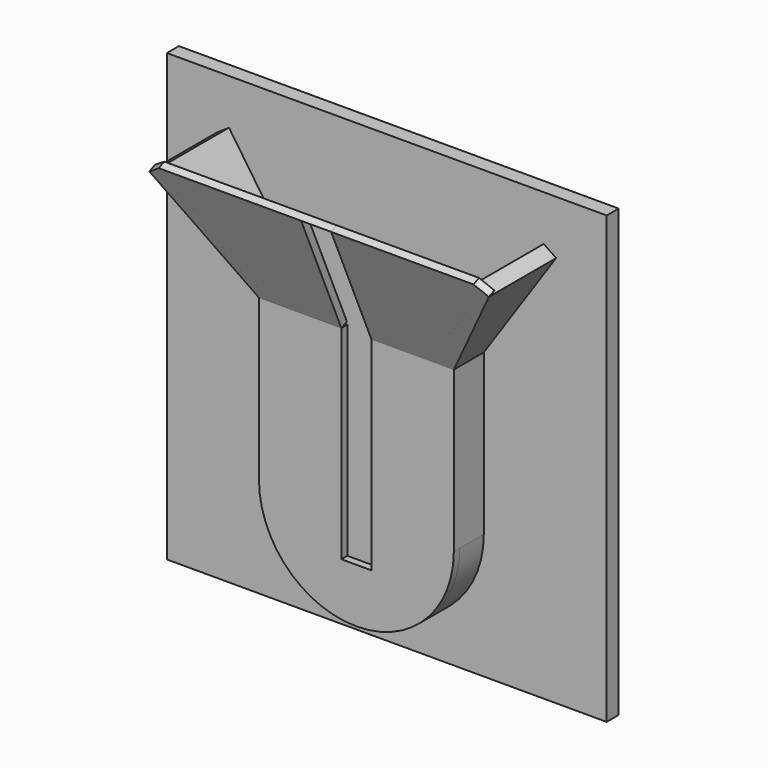
from build123d import *

# Parameters (mm, degrees)
F1_DEPTH     = 50.8
F2_W         = 745.3036904335
F2_H         = 755.5955052376
F3_DEPTH     = 25.4
F5_DEPTH     = 12.7
F7_DEPTH     = 101.6
F8_T4_DEPTH  = 1078.7585913979
F9_DEPTH     = 101.6
F10_T4_DEPTH = 1078.7585913979
F12_DEPTH    = 12.7


# Not quite as in the source:
# - a fillet or chamfer that OpenCascade refuses, or shapes differently, is made with other operations: its cross-section is extruded or revolved along the edge and cut away or added


with BuildPart() as f1:
    # F0 (on Front) → F1 (new body)
    with BuildSketch(Plane.XZ):
        with BuildLine():
            Line((-89.9567651826, 106.8080672332), (-216.9567651826, 293.8318768854))
            Line((-216.9567651826, 293.8318768854), (-237.969898878, 279.5627419326))
            Line((-237.969898878, 279.5627419326), (-216.9567651826, 248.6182040079))
            Line((-216.9567651826, 248.6182040079), (-115.3567651826, 98.9991562862))
            Line((-115.3567651826, 98.9991562862), (-115.3567651826, -172.5919327668))
            ThreePointArc((-115.3567651826, -172.5919327668), (-67.0000946798, -289.3352624173), (49.7432350342, -337.6919327668))
            ThreePointArc((49.7432350342, -337.6919327668), (166.486564468, -289.335262264), (214.8432348174, -172.5919327668))
            Line((214.8432348174, -172.5919327668), (214.8432348174, 98.9991562862))
            Line((214.8432348174, 98.9991562862), (316.4432348174, 248.6182040079))
            Line((316.4432348174, 248.6182040079), (337.4563685128, 279.5627419326))
            Line((337.4563685128, 279.5627419326), (316.4432348174, 293.8318768854))
            Line((316.4432348174, 293.8318768854), (189.4432348174, 106.8080672332))
            Line((189.4432348174, 106.8080672332), (189.4432348174, -172.5919327668))
            ThreePointArc((189.4432348174, -172.5919327668), (49.7432348174, -312.2919327668), (-89.9567651826, -172.5919327668))
            Line((-89.9567651826, -172.5919327668), (-89.9567651826, 106.8080672332))
        make_face()
    extrude(amount=F1_DEPTH)

    # F2 (on face) → F3 (join)
    with BuildSketch(Plane(origin=(0, 0, 0), x_dir=(-1, 0, 0), z_dir=(0, 1, 0))):
        with Locations((-50.4573881626, -6.8071186543)):
            Rectangle(F2_W, F2_H)
        with BuildLine():
            Line((89.9567651826, 106.8080672332), (216.9567651826, 293.8318768854))
            Line((216.9567651826, 293.8318768854), (237.969898878, 279.5627419326))
            Line((237.969898878, 279.5627419326), (115.3567651826, 98.9991562862))
            Line((115.3567651826, 98.9991562862), (115.3567651826, -172.5919327668))
            ThreePointArc((115.3567651826, -172.5919327668), (-49.7432348174, -337.6919327668), (-214.8432348174, -172.5919327668))
            Line((-214.8432348174, -172.5919327668), (-214.8432348174, 98.9991562862))
            Line((-214.8432348174, 98.9991562862), (-337.4563685128, 279.5627419326))
            Line((-337.4563685128, 279.5627419326), (-316.4432348174, 293.8318768854))
            Line((-316.4432348174, 293.8318768854), (-189.4432348174, 106.8080672332))
            Line((-189.4432348174, 106.8080672332), (-189.4432348174, -172.5919327668))
            ThreePointArc((-189.4432348174, -172.5919327668), (-49.7432348174, -312.2919327668), (89.9567651826, -172.5919327668))
            Line((89.9567651826, -172.5919327668), (89.9567651826, 106.8080672332))
        make_face(mode=Mode.SUBTRACT)
        with BuildLine():
            Line((237.969898878, 279.5627419326), (216.9567651826, 293.8318768854))
            Line((216.9567651826, 293.8318768854), (89.9567651826, 106.8080672332))
            Line((89.9567651826, 106.8080672332), (89.9567651826, -172.5919327668))
            ThreePointArc((89.9567651826, -172.5919327668), (-49.7432348174, -312.2919327668), (-189.4432348174, -172.5919327668))
            Line((-189.4432348174, -172.5919327668), (-189.4432348174, 106.8080672332))
            Line((-189.4432348174, 106.8080672332), (-316.4432348174, 293.8318768854))
            Line((-316.4432348174, 293.8318768854), (-337.4563685128, 279.5627419326))
            Line((-337.4563685128, 279.5627419326), (-214.8432348174, 98.9991562862))
            Line((-214.8432348174, 98.9991562862), (-214.8432348174, -172.5919327668))
            ThreePointArc((-214.8432348174, -172.5919327668), (-49.7432348174, -337.6919327668), (115.3567651826, -172.5919327668))
            Line((115.3567651826, -172.5919327668), (115.3567651826, 98.9991562862))
            Line((115.3567651826, 98.9991562862), (237.969898878, 279.5627419326))
        make_face()
    extrude(amount=F3_DEPTH)

    # F4 (on face) → F5 (join)
    with BuildSketch(Plane.XZ.offset(50.8)):
        with BuildLine():
            Line((24.3432348174, 98.9991562862), (-89.9567651826, 98.9991562862))
            Line((-89.9567651826, 98.9991562862), (-89.9567651826, -172.5919327668))
            ThreePointArc((-89.9567651826, -172.5919327668), (49.7432348174, -312.2919327668), (189.4432348174, -172.5919327668))
            Line((189.4432348174, -172.5919327668), (189.4432348174, 98.9991562862))
            Line((189.4432348174, 98.9991562862), (75.1432348174, 98.9991562862))
            Line((75.1432348174, 98.9991562862), (75.1432348174, -172.5919327668))
            Line((75.1432348174, -172.5919327668), (75.1432348174, -245.7823455334))
            Line((75.1432348174, -245.7823455334), (24.3432348174, -245.7823455334))
            Line((24.3432348174, -245.7823455334), (24.3432348174, -172.5919327668))
            Line((24.3432348174, -172.5919327668), (24.3432348174, 98.9991562862))
        make_face()
        with BuildLine():
            Line((-89.9567651826, -172.5919327668), (-89.9567651826, 98.9991562862))
            Line((-89.9567651826, 98.9991562862), (-115.3567651826, 98.9991562862))
            Line((-115.3567651826, 98.9991562862), (-115.3567651826, -172.5919327668))
            ThreePointArc((-115.3567651826, -172.5919327668), (49.7432348174, -337.6919327668), (214.8432348174, -172.5919327668))
            Line((214.8432348174, -172.5919327668), (214.8432348174, 98.9991562862))
            Line((214.8432348174, 98.9991562862), (189.4432348174, 98.9991562862))
            Line((189.4432348174, 98.9991562862), (189.4432348174, -172.5919327668))
            ThreePointArc((189.4432348174, -172.5919327668), (49.7432348174, -312.2919327668), (-89.9567651826, -172.5919327668))
        make_face()
    extrude(amount=F5_DEPTH)

    # F6 (on face) → F7 (join)
    with BuildSketch(Plane.XZ.offset(50.8)):
        Polygon((-118.501645235, 103.6303960366), (-115.3567651826, 98.9991562862), (-89.9567651826, 98.9991562862), (-89.9567651826, 106.8080672332), (-216.9567651826, 293.8318768854), (-237.969898878, 279.5627419326), align=None)
    extrude(amount=F7_DEPTH)

    # F8: chamfer of 88.9 x 203.2 on 1 edges, made by hand


with BuildPart() as f8_tool2:
    # F8_s3 → F8_t4 (new body)
    with BuildSketch(Plane.YZ.offset(-642.0360608816)):
        Polygon((-152.4, 302.1991562862), (-63.5, 98.9991562862), (-152.4, 98.9991562862), align=None)
    extrude(amount=F8_T4_DEPTH)

    split(bisect_by=Plane.XZ.offset(63.5), keep=Keep.TOP)


with BuildPart() as f1_1:
    add(f1.part)

    # F8_t1: cut F8_tool2
    add(f8_tool2.part, mode=Mode.SUBTRACT)

    # F9 (add): a face of the model
    f9_faces = [f1_1.faces().sort_by_distance(p)[0] for p in [
        (263.3288281635, -50.8, 193.2225963664),
    ]]
    extrude(f9_faces, amount=F9_DEPTH)

    # F10: chamfer of 203.2 x 88.9 on 1 edges, made by hand


with BuildPart() as f10_tool2:
    # F10_s3 → F10_t4 (new body)
    with BuildSketch(Plane.YZ.offset(741.5225305163)):
        Polygon((-63.5, 98.9991562862), (-152.4, 302.1991562862), (-152.4, 98.9991562862), align=None)
    extrude(amount=-F10_T4_DEPTH)

    split(bisect_by=Plane.XZ.offset(63.5), keep=Keep.TOP)


with BuildPart() as f1_2:
    add(f1_1.part)

    # F10_t1: cut F10_tool2
    add(f10_tool2.part, mode=Mode.SUBTRACT)


with BuildPart() as f12:
    # F11 (on face) → F12 (new body)
    with BuildSketch(Plane(origin=(0, -16.9445721179, -7.4132503016), x_dir=(1, 0, 0), z_dir=(0, -0.9161573349, -0.400818834))):
        Polygon((-237.969898878, 313.2387651133), (-115.3567651826, 116.150799141), (-89.9567651826, 116.150799141), (-89.9567651826, 124.6743470618), (-216.9567651826, 328.8137481529), align=None)
        Polygon((-89.9567651826, 124.6743470618), (-89.9567651826, 116.150799141), (24.3432348174, 116.150799141), (24.3432348174, 328.8111325348), (75.1432348174, 328.8111325348), (-216.9567651826, 328.8137481529), align=None)
    extrude(amount=-F12_DEPTH)


with BuildPart() as f12b:
    # F11 (on face) → F12, piece 2 (new body)
    with BuildSketch(Plane(origin=(0, -16.9445721179, -7.4132503016), x_dir=(1, 0, 0), z_dir=(0, -0.9161573349, -0.400818834))):
        Polygon((75.1432348174, 328.8111325348), (75.1432348174, 116.150799141), (214.8432348174, 116.150799141), (337.4563754174, 313.238771741), (316.4505754174, 328.808971741), align=None)
    extrude(amount=-F12_DEPTH)


solid = Compound([f1_2.part, f12.part, f12b.part])
